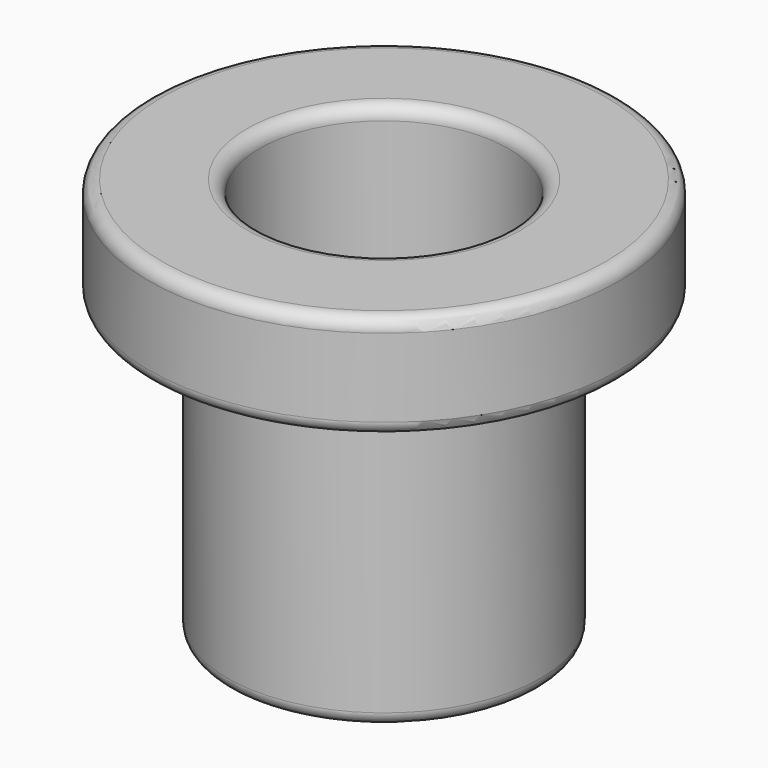
from build123d import *

# Parameters (mm, degrees)
F0_R     = 9
F1_DEPTH = 4
F2_R     = 6
F3_DEPTH = 11.35
F4_R     = 4.75
F5_DEPTH = 13.35
F6_R     = 0.5
F7_R     = 2.5
F8_DEPTH = 2.001
F9_R     = 0.5


# Not quite as in the source:
# - two fillets or chamfers of one size are made in one step


with BuildPart() as f1:
    # F0 (on Top) → F1 (new body)
    with BuildSketch(Plane.XY):
        Circle(F0_R)
    extrude(amount=F1_DEPTH)

    # F2 (on face) → F3 (join)
    with BuildSketch(Plane(origin=(0, 0, 0), x_dir=(1, 0, 0), z_dir=(0, 0, -1))):
        Circle(F2_R)
    extrude(amount=F3_DEPTH)

    # F4 (on face) → F5 (cut, through all)
    with BuildSketch(Plane.XY.offset(4)):
        Circle(F4_R)
    extrude(amount=-F5_DEPTH, mode=Mode.SUBTRACT)

    # F6
    f6_edges = [f1.edges().sort_by_distance(p)[0] for p in [
        (-9, 0, 4),
        (-6, 0, 0),
        (-9, 0, 0),
        (-4.75, 0, 4),
        (-6, 0, -11.35),
        (-4.75, 0, -9.35),
    ]]
    fillet(f6_edges, radius=F6_R)

    # F7 (on face) → F8 (cut, through all)
    with BuildSketch(Plane.XY.offset(-9.35)):
        Circle(F7_R)
    extrude(amount=-F8_DEPTH, mode=Mode.SUBTRACT)

    # F9
    f9_edges = [f1.edges().sort_by_distance(p)[0] for p in [
        (-2.5, 0, -11.35),
        (-2.5, 0, -9.35),
    ]]
    fillet(f9_edges, radius=F9_R)


solid = f1.part
